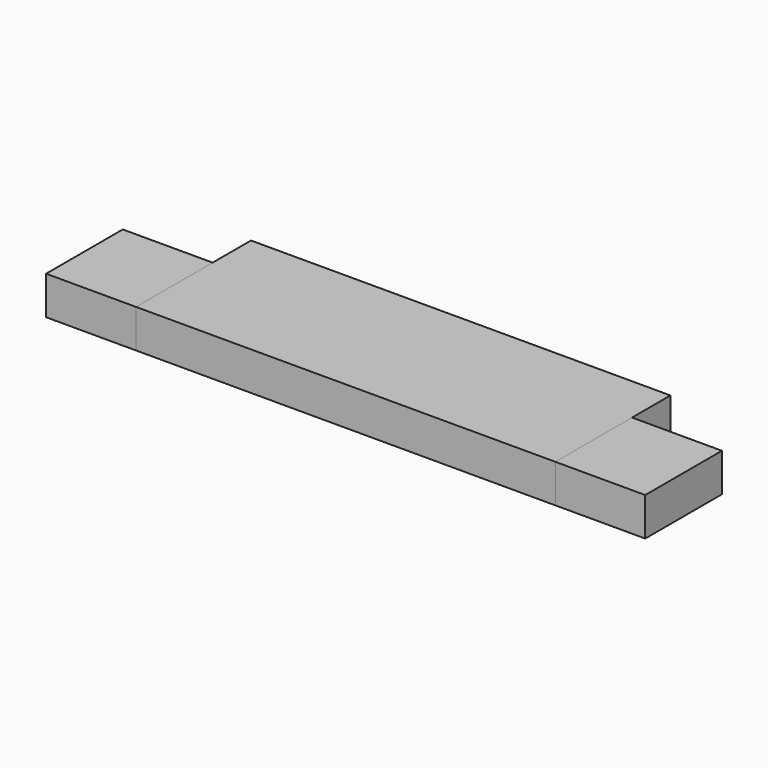
from build123d import *

# Parameters (mm, degrees)
F0_W     = 17.5
F0_H     = 4
F1_DEPTH = 1.6
F0_W_2   = 3.75
F2_DEPTH = 1.6
F3_DEPTH = 2


with BuildPart() as f1:
    # F0 (on Top) → F1 (new body)
    with BuildSketch(Plane.XY):
        Rectangle(F0_W, F0_H)
    extrude(amount=F1_DEPTH)

    # F3 (add): a face of the model
    f3_faces = [f1.faces().sort_by_distance(p)[0] for p in [
        (0, 2, 0.8),
    ]]
    extrude(f3_faces, amount=F3_DEPTH)


with BuildPart() as f2:
    # F0 (on Top) → F2 (new body, through all)
    with BuildSketch(Plane.XY):
        with Locations((-10.625, 0)):
            Rectangle(F0_W_2, F0_H)
    extrude(amount=F2_DEPTH)


with BuildPart() as f2b:
    # F0 (on Top) → F2, piece 2 (new body, through all)
    with BuildSketch(Plane.XY):
        with Locations((10.625, 0)):
            Rectangle(F0_W_2, F0_H)
    extrude(amount=F2_DEPTH)


solid = Compound([f1.part, f2.part, f2b.part])
